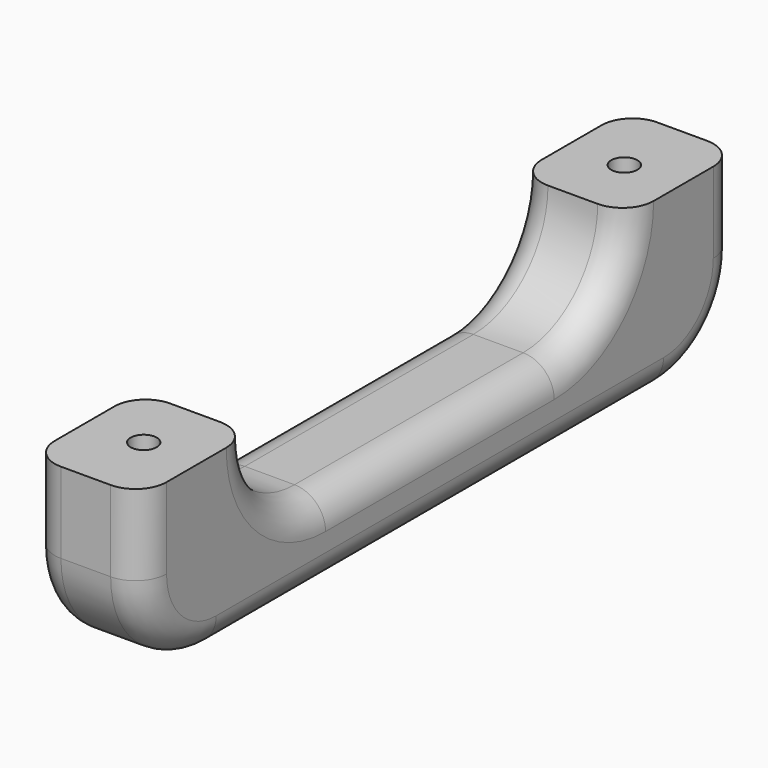
from build123d import *

# Parameters (mm, degrees)
F1_DEPTH     = 18
F3_R         = 2.1
F4_DEPTH     = 25
F5_R         = 14.99999
F6_T1_DEPTH  = 90.00002
F6_T3_DEPTH  = 46.00002
F6_T5_DEPTH  = 12.50001
F6_T7_DEPTH  = 25.50001
F6_T10_ANGLE = 90
F6_T12_ANGLE = 90
F6_T14_ANGLE = 90
F6_T16_ANGLE = 90
F6_T18_ANGLE = 90
F6_T20_ANGLE = 90
F6_T22_ANGLE = 90
F6_T24_ANGLE = 90


# Not quite as in the source:
# - a fillet or chamfer that OpenCascade refuses, or shapes differently, is made with other operations: its cross-section is extruded or revolved along the edge and cut away or added
# - a fillet or chamfer is up to 0.001 mm smaller than in the source, because OpenCascade refuses the exact size


with BuildPart() as f1:
    # F0 (on Right) → F1 (new body)
    with BuildSketch(Plane.YZ):
        Polygon((-60, 28), (-60, 0), (0, 0), (60, 0), (60, 28), (38, 28), (38, 13), (-38, 13), (-38, 28), align=None)
    extrude(amount=F1_DEPTH)

    # F3 (on offset) → F4 (cut)
    with BuildSketch(Plane.XY.offset(28)):
        with Locations((9, 48.35)):
            Circle(F3_R)
        with Locations((9, -48.35)):
            Circle(F3_R)
    extrude(amount=-F4_DEPTH, mode=Mode.SUBTRACT)

    # F5 (radius 15 in the source; OpenCascade refuses exactly that, so slightly less here)
    f5_edges = [f1.edges().sort_by_distance(p)[0] for p in [
        (9, 60, 0),
        (9, -60, 0),
        (9, -38, 13),
        (9, 38, 13),
    ]]
    fillet(f5_edges, radius=F5_R)

    # F6: fillet of radius 5 on 4 edges, made by hand

    # F6_s2 → F6_t1 (cut)
    with BuildSketch(Plane.XZ.offset(-45.00001)):
        with BuildLine():
            ThreePointArc((0, 5), (1.4644660941, 1.4644660941), (5, 0))
            Line((5, 0), (0, 0))
            Line((0, 0), (0, 5))
        make_face()
        with BuildLine():
            ThreePointArc((18, 5), (16.5355339059, 1.4644660941), (13, 0))
            Line((13, 0), (18, 0))
            Line((18, 0), (18, 5))
        make_face()
    extrude(amount=F6_T1_DEPTH, mode=Mode.SUBTRACT)

    # F6_s4 → F6_t3 (cut)
    with BuildSketch(Plane.XZ.offset(-23.00001)):
        with BuildLine():
            ThreePointArc((0, 8), (1.4644660941, 11.5355339059), (5, 13))
            Line((5, 13), (0, 13))
            Line((0, 13), (0, 8))
        make_face()
        with BuildLine():
            ThreePointArc((18, 8), (16.5355339059, 11.5355339059), (13, 13))
            Line((13, 13), (18, 13))
            Line((18, 13), (18, 8))
        make_face()
    extrude(amount=F6_T3_DEPTH, mode=Mode.SUBTRACT)

    # F6_s6 → F6_t5 (cut)
    with BuildSketch(Plane.XY.offset(27.99999)):
        with BuildLine():
            ThreePointArc((18, -43), (16.5355339059, -39.4644660941), (13, -38))
            Line((13, -38), (18, -38))
            Line((18, -38), (18, -43))
        make_face()
        with BuildLine():
            ThreePointArc((18, 43), (16.5355339059, 39.4644660941), (13, 38))
            Line((13, 38), (18, 38))
            Line((18, 38), (18, 43))
        make_face()
        with BuildLine():
            ThreePointArc((0, -43), (1.4644660941, -39.4644660941), (5, -38))
            Line((5, -38), (0, -38))
            Line((0, -38), (0, -43))
        make_face()
        with BuildLine():
            ThreePointArc((0, 43), (1.4644660941, 39.4644660941), (5, 38))
            Line((5, 38), (0, 38))
            Line((0, 38), (0, 43))
        make_face()
    extrude(amount=F6_T5_DEPTH, mode=Mode.SUBTRACT)

    # F6_s8 → F6_t7 (cut)
    with BuildSketch(Plane.XY.offset(14.99999)):
        with BuildLine():
            ThreePointArc((13, -60), (16.5355339059, -58.5355339059), (18, -55))
            Line((18, -55), (18, -60))
            Line((18, -60), (13, -60))
        make_face()
        with BuildLine():
            ThreePointArc((18, 55), (16.5355339059, 58.5355339059), (13, 60))
            Line((13, 60), (18, 60))
            Line((18, 60), (18, 55))
        make_face()
        with BuildLine():
            ThreePointArc((0, 55), (1.4644660941, 58.5355339059), (5, 60))
            Line((5, 60), (0, 60))
            Line((0, 60), (0, 55))
        make_face()
        with BuildLine():
            ThreePointArc((5, -60), (1.4644660941, -58.5355339059), (0, -55))
            Line((0, -55), (0, -60))
            Line((0, -60), (5, -60))
        make_face()
    extrude(amount=F6_T7_DEPTH, mode=Mode.SUBTRACT)

    # F6_s9 → F6_t10 (revolve, cut)
    with BuildSketch(Plane.XY.offset(27.99999)):
        with BuildLine():
            ThreePointArc((18, 43), (16.5355339059, 39.4644660941), (13, 38))
            Line((13, 38), (18, 38))
            Line((18, 38), (18, 43))
        make_face()
    revolve(axis=Axis((18, 23.00001, 27.99999), (-1, 0, 0)), revolution_arc=F6_T10_ANGLE, mode=Mode.SUBTRACT)

    # F6_s11 → F6_t12 (revolve, cut)
    with BuildSketch(Plane.XY.offset(27.99999)):
        with BuildLine():
            ThreePointArc((18, -43), (16.5355339059, -39.4644660941), (13, -38))
            Line((13, -38), (18, -38))
            Line((18, -38), (18, -43))
        make_face()
    revolve(axis=Axis((18, -23.00001, 27.99999), (1, 0, 0)), revolution_arc=F6_T12_ANGLE, mode=Mode.SUBTRACT)

    # F6_s13 → F6_t14 (revolve, cut)
    with BuildSketch(Plane.XY.offset(27.99999)):
        with BuildLine():
            ThreePointArc((0, 43), (1.4644660941, 39.4644660941), (5, 38))
            Line((5, 38), (0, 38))
            Line((0, 38), (0, 43))
        make_face()
    revolve(axis=Axis((0, 23.00001, 27.99999), (-1, 0, 0)), revolution_arc=F6_T14_ANGLE, mode=Mode.SUBTRACT)

    # F6_s15 → F6_t16 (revolve, cut)
    with BuildSketch(Plane.XY.offset(27.99999)):
        with BuildLine():
            ThreePointArc((0, -43), (1.4644660941, -39.4644660941), (5, -38))
            Line((5, -38), (0, -38))
            Line((0, -38), (0, -43))
        make_face()
    revolve(axis=Axis((0, -23.00001, 27.99999), (1, 0, 0)), revolution_arc=F6_T16_ANGLE, mode=Mode.SUBTRACT)

    # F6_s17 → F6_t18 (revolve, cut)
    with BuildSketch(Plane.XZ.offset(-45.00001)):
        with BuildLine():
            ThreePointArc((18, 5), (16.5355339059, 1.4644660941), (13, 0))
            Line((13, 0), (18, 0))
            Line((18, 0), (18, 5))
        make_face()
    revolve(axis=Axis((18, 45.00001, 14.99999), (1, 0, 0)), revolution_arc=F6_T18_ANGLE, mode=Mode.SUBTRACT)

    # F6_s19 → F6_t20 (revolve, cut)
    with BuildSketch(Plane.XY.offset(14.99999)):
        with BuildLine():
            ThreePointArc((13, -60), (16.5355339059, -58.5355339059), (18, -55))
            Line((18, -55), (18, -60))
            Line((18, -60), (13, -60))
        make_face()
    revolve(axis=Axis((18, -45.00001, 14.99999), (1, 0, 0)), revolution_arc=F6_T20_ANGLE, mode=Mode.SUBTRACT)

    # F6_s21 → F6_t22 (revolve, cut)
    with BuildSketch(Plane.XY.offset(14.99999)):
        with BuildLine():
            ThreePointArc((0, -55), (1.4644660941, -58.5355339059), (5, -60))
            Line((5, -60), (0, -60))
            Line((0, -60), (0, -55))
        make_face()
    revolve(axis=Axis((0, -45.00001, 14.99999), (1, 0, 0)), revolution_arc=F6_T22_ANGLE, mode=Mode.SUBTRACT)

    # F6_s23 → F6_t24 (revolve, cut)
    with BuildSketch(Plane.XZ.offset(-45.00001)):
        with BuildLine():
            ThreePointArc((0, 5), (1.4644660941, 1.4644660941), (5, 0))
            Line((5, 0), (0, 0))
            Line((0, 0), (0, 5))
        make_face()
    revolve(axis=Axis((0, 45.00001, 14.99999), (1, 0, 0)), revolution_arc=F6_T24_ANGLE, mode=Mode.SUBTRACT)


solid = f1.part
